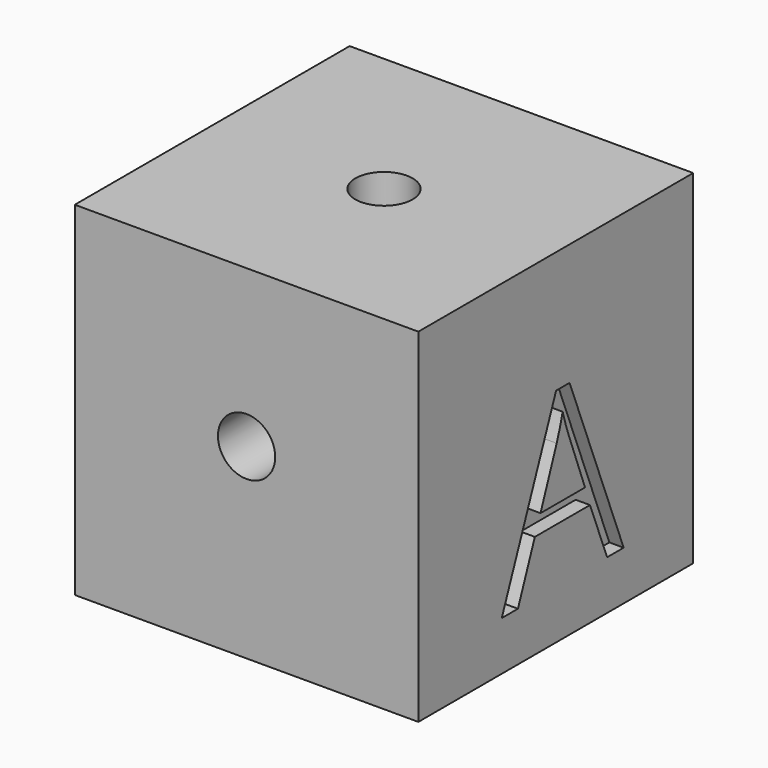
from build123d import *

# Parameters (mm, degrees)
F0_W          = 19.05
F0_H          = 19.05
F1_DEPTH      = 19.05
F2_R          = 1.5875
F3_DEPTH      = 25.4
F4_R          = 1.5875
F5_DEPTH      = 6.35
F6_TEXT_SIZE  = 13.3534990406
F7_DEPTH      = 0.79375
F8_TEXT_SIZE  = 16.7406280525
F9_DEPTH      = 0.79375
F10_TEXT_SIZE = 17.0059206236
F11_DEPTH     = 0.79375


# Not quite as in the source:
# - a length typed as a fraction of an inch, garbled in the dataset ("3 / 203.2 mm" for 3/8 in), is restored
# - Text() gives the source's letters only with a copy of the font that has no kerning and outlines rounded to 1/6400 em; it was checked with that copy


with BuildPart() as f1:
    # F0 (on Top) → F1 (new body)
    with BuildSketch(Plane.XY):
        Rectangle(F0_W, F0_H)
    extrude(amount=F1_DEPTH)

    # F2 (on face) → F3 (cut)
    with BuildSketch(Plane.XY):
        Circle(F2_R)
    extrude(amount=F3_DEPTH, mode=Mode.SUBTRACT)

    # F4 (on face) → F5 (cut)
    with BuildSketch(Plane.XZ.offset(9.525)):
        with Locations((0, 10.3457062982)):
            Circle(F4_R)
    extrude(amount=-F5_DEPTH, mode=Mode.SUBTRACT)

    # F6 (on face) → F7 (cut)
    with BuildSketch(Plane.YZ.offset(9.525)):
        with Locations((-3.7451393437, 2.7190153487)):
            Text('A', F6_TEXT_SIZE, font='Open Sans', text_align=(TextAlign.LEFT, TextAlign.BOTTOM))
    extrude(amount=-F7_DEPTH, mode=Mode.SUBTRACT)

    # F8 (on face) → F9 (cut)
    with BuildSketch(Plane(origin=(0, 9.525, 0), x_dir=(-1, 0, 0), z_dir=(0, 1, 0))):
        with Locations((-5.4387357086, 1.6402490437)):
            Text('R', F8_TEXT_SIZE, font='Open Sans', text_align=(TextAlign.LEFT, TextAlign.BOTTOM))
    extrude(amount=-F9_DEPTH, mode=Mode.SUBTRACT)

    # F10 (on face) → F11 (cut)
    with BuildSketch(Plane(origin=(-9.525, 0, 0), x_dir=(0, -1, 0), z_dir=(-1, 0, 0))):
        with Locations((-5.9030377306, 1.3510443969)):
            Text('S', F10_TEXT_SIZE, font='Open Sans', text_align=(TextAlign.LEFT, TextAlign.BOTTOM))
    extrude(amount=-F11_DEPTH, mode=Mode.SUBTRACT)


solid = f1.part
